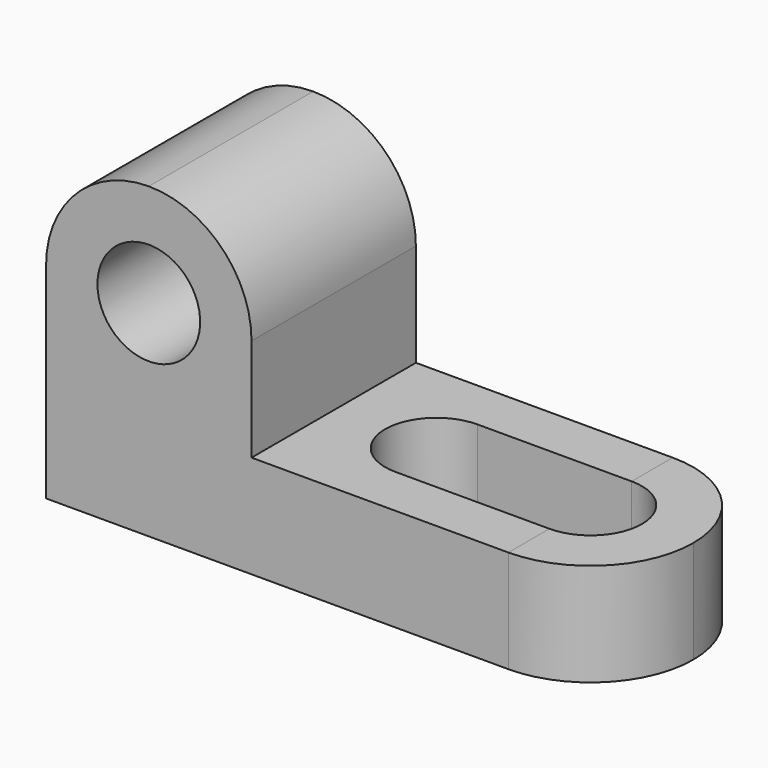
from build123d import *

# Parameters (mm, degrees)
F1_DEPTH = 25.4
F3_DEPTH = 12.7
F5_D     = 12.7
F7_DEPTH = 25.4


# Not quite as in the source:
# - ends of sketch curves that miss each other by under 0.0002 mm in the source are joined


with BuildPart() as f1:
    # F0 (on Front) → F1 (new body)
    with BuildSketch(Plane.XZ):
        Polygon((-70.2426877682, 36.4766385419), (-82.9426877682, 36.4766391127), (-82.9426877682, 11.0766391127), (-25.7926877682, 11.0766391127), (-25.7926877682, 23.776637971), (-57.5426877682, 23.776637971), (-57.5426877682, 36.476637971), align=None)
        with BuildLine():
            Line((-70.2426871973, 49.176637971), (-70.2426877682, 36.476637971))
            Line((-70.2426877682, 36.476637971), (-57.5426877682, 36.476637971))
            ThreePointArc((-57.5426877682, 36.476637971), (-61.2624314453, 45.4568938903), (-70.2426871973, 49.176637971))
        make_face()
        with BuildLine():
            ThreePointArc((-70.2426871973, 49.176637971), (-79.2229432838, 45.4568946976), (-82.9426877682, 36.4766391127))
            Line((-82.9426877682, 36.4766391127), (-70.2426877682, 36.4766385419))
            Line((-70.2426877682, 36.4766385419), (-70.2426871973, 49.176637971))
        make_face()
    extrude(amount=F1_DEPTH)

    # F5 (through all)
    with Locations(Plane.XZ.offset(25.4)):
        with Locations((-70.2426877682, 36.476637971)):
            Hole(F5_D / 2)


with BuildPart() as f3:
    # F2 (on face) → F3 (new body)
    with BuildSketch(Plane.XY.offset(23.776637971)):
        with BuildLine():
            Line((-25.7926877682, -12.7), (-13.0926877682, -12.7))
            ThreePointArc((-13.0926877682, -12.7), (-16.8124316471, -3.7197438789), (-25.7926877682, 0))
            Line((-25.7926877682, 0), (-25.7926877682, -12.7))
        make_face()
        with BuildLine():
            Line((-25.7926877682, -12.7), (-25.7926877682, -25.4))
            ThreePointArc((-25.7926877682, -25.4), (-16.8124316471, -21.6802561211), (-13.0926877682, -12.7))
            Line((-13.0926877682, -12.7), (-25.7926877682, -12.7))
        make_face()
    extrude(amount=-F3_DEPTH)


with BuildPart() as f7_tool:
    # F6 (on face) → F7 (new body)
    with BuildSketch(Plane.XY.offset(23.776637971)):
        with BuildLine():
            ThreePointArc((-25.7926877682, -19.0500009306), (-19.4426877682, -12.7000009306), (-25.7926877682, -6.3500009306))
            Line((-25.7926877682, -6.3500009306), (-25.7926877682, -19.0500009306))
        make_face()
        Polygon((-25.7926877682, -6.3500009306), (-44.8426877682, -6.35), (-44.8426877682, -19.0500009306), (-25.7926877682, -19.0500009306), align=None)
        with BuildLine():
            Line((-44.8426877682, -19.0500009306), (-44.8426877682, -6.35))
            ThreePointArc((-44.8426877682, -6.35), (-51.1926885437, -12.7000004653), (-44.8426877682, -19.0500009306))
        make_face()
    extrude(amount=-F7_DEPTH)


with BuildPart() as f1_1:
    add(f1.part)

    # F7: cut by f7_tool
    add(f7_tool.part, mode=Mode.SUBTRACT)


with BuildPart() as f3_1:
    add(f3.part)

    # F7: cut by f7_tool
    add(f7_tool.part, mode=Mode.SUBTRACT)


solid = Compound([f1_1.part, f3_1.part])
